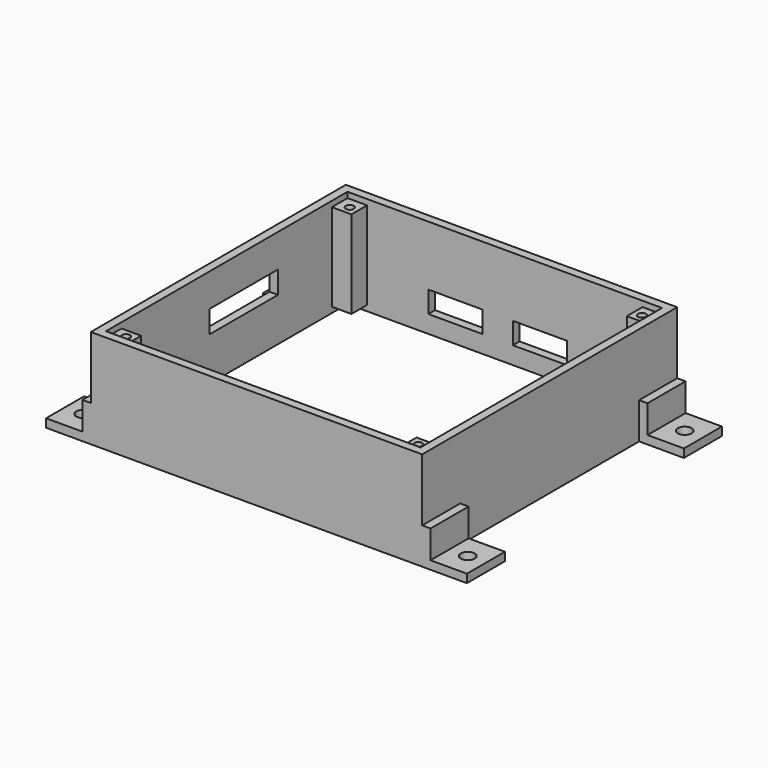
from build123d import *

# Parameters (mm, degrees)
F0_W      = 118.5
F0_H      = 114
F0_W_2    = 112.5
F0_H_2    = 108
F1_DEPTH  = 35.36
F3_START  = -2
F2_W      = 7
F2_H      = 7
F3_DEPTH  = 31.36
F4_R      = 1.45
F5_DEPTH  = 33.361
F6_W      = 30.51
F6_H      = 8
F7_DEPTH  = 3
F8_W      = 19.4
F8_H      = 7.7
F9_DEPTH  = 3
F11_DEPTH = 114
F13_DEPTH = 114
F15_W     = 16
F15_H     = 80
F16_DEPTH = 35.361
F17_W     = 16
F17_H     = 80
F18_DEPTH = 35.361
F19_R     = 2.5
F20_DEPTH = 3.001


# Not quite as in the source:
# - a feature names something its author has since deleted; it is built from what else it names


with BuildPart() as f1:
    # F0 (on Top) → F1 (new body)
    with BuildSketch(Plane.XY):
        with Locations((56.25, 54)):
            Rectangle(F0_W, F0_H)
        with Locations((56.25, 54)):
            Rectangle(F0_W_2, F0_H_2, mode=Mode.SUBTRACT)
    extrude(amount=F1_DEPTH)

    # F2 (on face) → F3 (join)
    with BuildSketch(Plane.XY.offset(35.36).offset(F3_START)):
        with Locations((3.5, 104.5)):
            Rectangle(F2_W, F2_H)
        with Locations((109, 104.5)):
            Rectangle(F2_W, F2_H)
        with Locations((109, 3.5)):
            Rectangle(F2_W, F2_H)
        with Locations((3.5, 3.5)):
            Rectangle(F2_W, F2_H)
    extrude(amount=-F3_DEPTH)

    # F4 (on face) → F5 (cut, through all)
    with BuildSketch(Plane.XY.offset(33.36)):
        with Locations((4, 104)):
            Circle(F4_R)
        with Locations((108.5, 104)):
            Circle(F4_R)
        with Locations((4, 4)):
            Circle(F4_R)
        with Locations((108.5, 4)):
            Circle(F4_R)
    extrude(amount=-F5_DEPTH, mode=Mode.SUBTRACT)

    # F6 (on face) → F7 (cut, through all)
    with BuildSketch(Plane(origin=(-3, 0, 0), x_dir=(0, -1, 0), z_dir=(-1, 0, 0))):
        with Locations((-61.615, 19.54)):
            Rectangle(F6_W, F6_H)
    extrude(amount=-F7_DEPTH, mode=Mode.SUBTRACT)

    # F8 (on face) → F9 (cut)
    with BuildSketch(Plane(origin=(0, 111, 0), x_dir=(-1, 0, 0), z_dir=(0, 1, 0))):
        with Locations((-68.83, 10.11)):
            Rectangle(F8_W, F8_H)
        with Locations((-38.62, 10.11)):
            Rectangle(F8_W, F8_H)
    extrude(amount=-F9_DEPTH, mode=Mode.SUBTRACT)

    # F10 (on face) → F11 (join)
    with BuildSketch(Plane.XZ.offset(3)):
        Polygon((-6, 3), (-19, 3), (-19, 0), (-3, 0), (-3, 13), (-6, 13), align=None)
    extrude(amount=-F11_DEPTH)

    # F12 (on face) → F13 (join)
    with BuildSketch(Plane.XZ.offset(3)):
        Polygon((118.5, 13), (115.5, 13), (115.5, 0), (131.5, 0), (131.5, 3), (118.5, 3), align=None)
    extrude(amount=-F13_DEPTH)

    # F15 (on face) → F16 (cut, through all)
    with BuildSketch(Plane(origin=(0, 0, 0), x_dir=(1, 0, 0), z_dir=(0, 0, -1))):
        with Locations((-11, -54)):
            Rectangle(F15_W, F15_H)
    extrude(amount=-F16_DEPTH, mode=Mode.SUBTRACT)

    # F17 (on face) → F18 (cut, through all)
    with BuildSketch(Plane(origin=(0, 0, 0), x_dir=(1, 0, 0), z_dir=(0, 0, -1))):
        with Locations((123.5, -54)):
            Rectangle(F17_W, F17_H)
    extrude(amount=-F18_DEPTH, mode=Mode.SUBTRACT)

    # F19 (on face) → F20 (cut, through all)
    with BuildSketch(Plane.XY.offset(3)):
        with Locations((-12.5, 102.5)):
            Circle(F19_R)
        with Locations((125, 102.5)):
            Circle(F19_R)
        with Locations((125, 5.5)):
            Circle(F19_R)
        with Locations((-12.5, 5.5)):
            Circle(F19_R)
    extrude(amount=-F20_DEPTH, mode=Mode.SUBTRACT)


solid = f1.part
